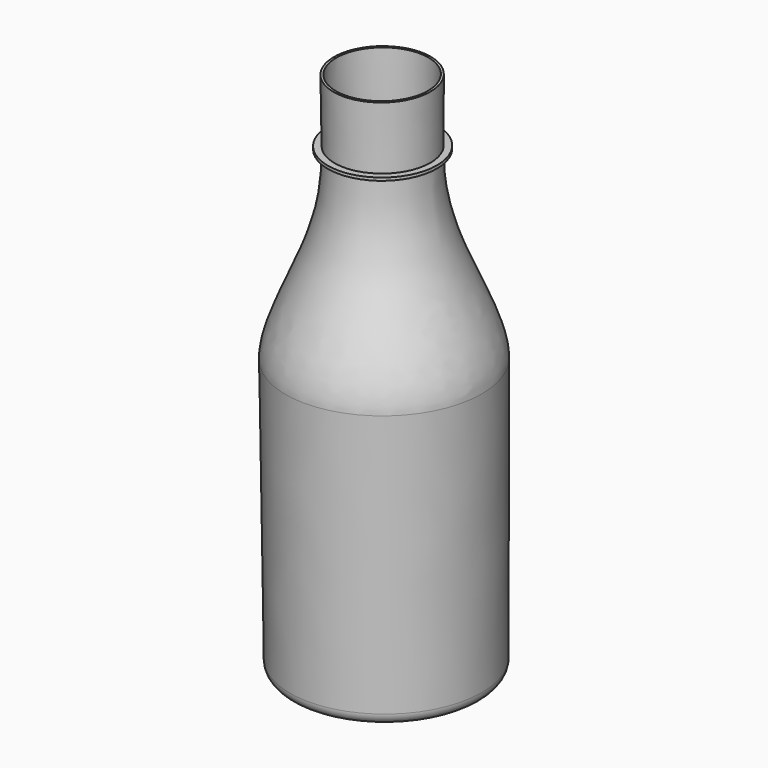
from build123d import *

# Parameters (mm, degrees)
F0_W = 2.1742532432
F0_H = 0.9419020339


# Not quite as in the source:
# - ends of sketch curves that miss each other by under 0.0002 mm in the source are joined
# - the dataset's text gives a spline's control points without its knots; the knots are read off the source's solid


with BuildPart() as f1:
    # F0 (on Front) → F1 (revolve)
    with BuildSketch(Plane.XZ):
        with BuildLine():
            Line((30.5, 90), (30.5, 4.1842871582))
            ThreePointArc((30.5, 4.1842871582), (29.2386865937, 1.7395031332), (26.5153540474, 1.3504783524))
            add(Edge.make_bspline(
                [(28.6535172577, 0.6161086402), (27.9351354208, 0.8594614999), (27.2238062641, 1.1043168589), (26.5153540474, 1.3504783524)],
                knots=[0.0654689301, 0.0654689301, 0.0654689301, 0.0654689301, 0.1426249603, 0.1426249603, 0.1426249603, 0.1426249603], degree=3))
            ThreePointArc((28.6535172577, 0.6161086402), (30.5321765876, 1.9778408883), (31.25, 4.1842871582))
            Line((31.25, 4.1842871582), (31.25, 90.000003855))
            add(Edge.make_bspline(
                [(31.25, 90.000003855), (31.2499948057, 91.0105522306), (31.0401649353, 93.1352024306), (29.9495012867, 97.7430729313), (27.5987257036, 104.0623990971), (24.0115192635, 112.0918752945), (20.4584738513, 120.0703885968), (17.7582794948, 127.4728481178), (15.2441676605, 137.0543853988), (14.4983428208, 144.4691488625), (14.4499999999, 150.0032696799)],
                knots=[0, 0, 0, 0, 0.0625, 0.125, 0.25, 0.375, 0.5, 0.625, 0.75, 0.9999509591, 0.9999509591, 0.9999509591, 0.9999509591], degree=3))
            Line((14.45, 150.0032696799), (14.45, 150.9451717138))
            Line((14.45, 150.9451717138), (14.45, 171.3955121697))
            Line((14.45, 171.3955121697), (13.7, 171.3955121697))
            Line((13.7, 171.3955121697), (13.7, 150))
            add(Edge.make_bspline(
                [(30.5, 90), (30.4999601958, 97.7439469245), (17.5798622294, 121.2385566117), (13.7960969357, 138.9584630881), (13.7, 150)],
                knots=[0, 0, 0, 0, 0.5049991048, 1, 1, 1, 1], degree=3))
        make_face()
        with BuildLine():
            add(Edge.make_bspline(
                [(28.6535172577, 0.6161086402), (27.9351354208, 0.8594614999), (27.2238062641, 1.1043168589), (26.5153540474, 1.3504783524)],
                knots=[0.0654689301, 0.0654689301, 0.0654689301, 0.0654689301, 0.1426249603, 0.1426249603, 0.1426249603, 0.1426249603], degree=3))
            add(Edge.make_bspline(
                [(26.5153540474, 1.3504783524), (23.505060911, 2.3964462197), (15.7684223832, 5.1935195764), (6.1960769817, 8.0488463864), (0, 8)],
                knots=[0.1426249603, 0.1426249603, 0.1426249603, 0.1426249603, 0.4704696092, 1, 1, 1, 1], degree=3))
            Line((0, 8), (0.0059123945, 7.2500233046))
            add(Edge.make_bspline(
                [(26.2691917605, 0.6420238521), (25.2813726049, 0.9852492871), (23.1576852685, 1.73281816), (20.4345242005, 2.6915237158), (18.0535614936, 3.508219), (15.6035591078, 4.32926986), (12.4109579359, 5.3369129826), (7.0731993079, 6.7140944287), (2.8622270402, 7.272540883), (0.0059123945, 7.2500233046)],
                knots=[0.1426251828, 0.1426251828, 0.1426251828, 0.1426251828, 0.25, 0.375, 0.4375, 0.5, 0.625, 0.75, 1, 1, 1, 1], degree=3))
            ThreePointArc((26.2691917605, 0.6420238521), (27.4592400633, 0.4345086811), (28.6535172577, 0.6161086402))
        make_face()
        with Locations((15.5371266216, 150.4742206969)):
            Rectangle(F0_W, F0_H)
    revolve(axis=Axis((0.0029561972, 0, 7.6250116523), (0.0078831927, 0, -0.9999689272)))


solid = f1.part
